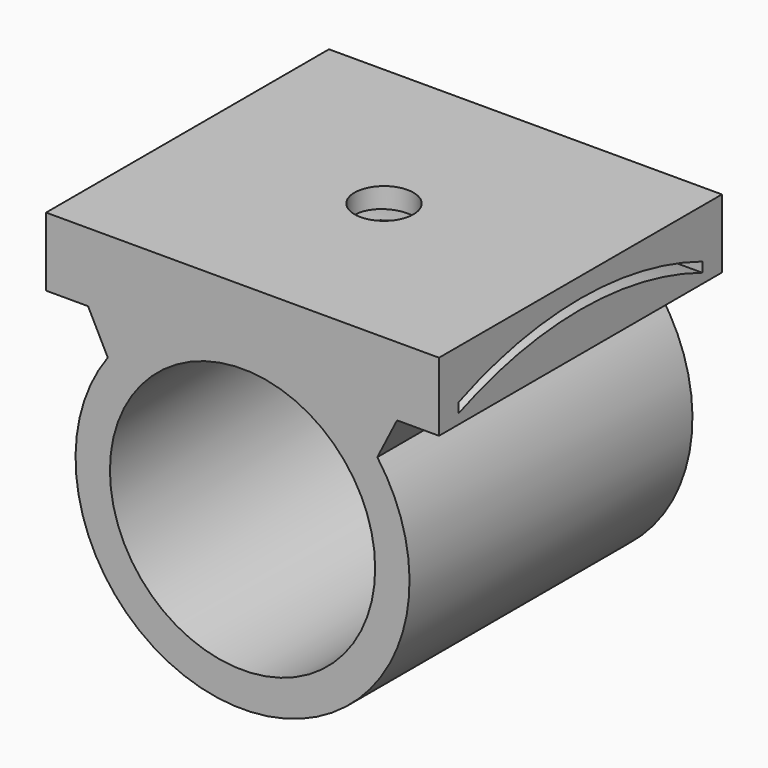
from build123d import *

# Parameters (mm, degrees)
F0_R         = 8.5
F1_DEPTH     = 18
F2_R         = 6.75
F3_DEPTH     = 18
F4_W         = 18
F4_H         = 3.5
F5_DEPTH     = 10
F7_DEPTH     = 20
F8_R         = 1.5
F9_DEPTH     = 5
F10_T1_DEPTH = 18


# Not quite as in the source:
# - a fillet or chamfer that OpenCascade refuses, or shapes differently, is made with other operations: its cross-section is extruded or revolved along the edge and cut away or added


with BuildPart() as f1:
    # F0 (on Front) → F1 (new body)
    with BuildSketch(Plane.XZ):
        Circle(F0_R)
    extrude(amount=F1_DEPTH)

    # F2 (on face) → F3 (cut, through all)
    with BuildSketch(Plane.XZ.offset(18)):
        Circle(F2_R)
    extrude(amount=-F3_DEPTH, mode=Mode.SUBTRACT)

    # F4 (on Right) → F5 (join, symmetric)
    with BuildSketch(Plane.YZ):
        with Locations((-9, 8.75)):
            Rectangle(F4_W, F4_H)
    extrude(amount=F5_DEPTH, both=True)

    # F6 (on face) → F7 (cut, through all)
    with BuildSketch(Plane.YZ.offset(10)):
        with BuildLine():
            Line((-16.75, 8), (-16.75, 7.5))
            ThreePointArc((-16.75, 7.5), (-9, 9), (-1.25, 7.5))
            Line((-1.25, 7.5), (-1.25, 8))
            ThreePointArc((-1.25, 8), (-9, 9.5), (-16.75, 8))
        make_face()
    extrude(amount=-F7_DEPTH, mode=Mode.SUBTRACT)

    # F8 (on face) → F9 (cut)
    with BuildSketch(Plane.XY.offset(10.5)):
        with Locations((0, -9)):
            Circle(F8_R)
    extrude(amount=-F9_DEPTH, mode=Mode.SUBTRACT)

    # F10: chamfer of 4 on 2 edges, made by hand

    # F10_s2 → F10_t1 (join)
    with BuildSketch(Plane.XZ):
        with BuildLine():
            Line((-6.7863990228, 4.8779762725), (-7.9352464288, 7.1426903404))
            Line((-7.9352464288, 7.1426903404), (-7.9352464288, 7.2226903404))
            ThreePointArc((-7.9352464288, 7.2226903404), (-6.3785359046, 7.08), (-4.8218253805, 7.08))
            Line((-4.8218253805, 7.08), (-4.7764434946, 6.9341176471))
            ThreePointArc((-4.7764434946, 6.9341176471), (-5.8850678371, 6.0218250184), (-6.7218457694, 4.8307229397))
            Line((-6.7218457694, 4.8307229397), (-6.7863990228, 4.8779762725))
        make_face()
        with BuildLine():
            Line((6.7863990228, 4.8779762725), (7.9352464288, 7.1426903404))
            Line((7.9352464288, 7.1426903404), (7.9352464288, 7.2226903404))
            ThreePointArc((7.9352464288, 7.2226903404), (6.3785359046, 7.08), (4.8218253805, 7.08))
            Line((4.8218253805, 7.08), (4.7764434946, 6.9341176471))
            ThreePointArc((4.7764434946, 6.9341176471), (5.8850678371, 6.0218250184), (6.7218457694, 4.8307229397))
            Line((6.7218457694, 4.8307229397), (6.7863990228, 4.8779762725))
        make_face()
    extrude(amount=F10_T1_DEPTH)


solid = f1.part
